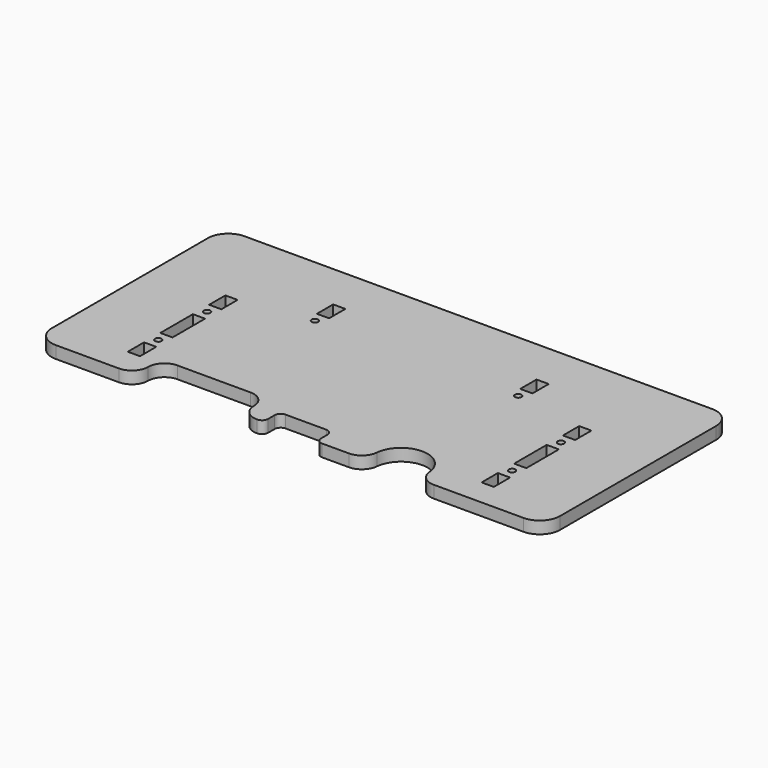
from build123d import *

# Parameters (mm, degrees)
F0_W     = 250
F0_H     = 116
F1_DEPTH = 6
F2_W     = 6
F2_H     = 10
F2_H_2   = 20
F2_W_2   = 26
F2_R     = 1.6
F2_W_3   = 52
F2_H_3   = 16
F3_DEPTH = 6.001
F4_R     = 3
F5_R     = 10
F6_R     = 7.99999
F7_R     = 1.6
F7_W     = 6
F7_H     = 10
F8_DEPTH = 6.0010001


# Not quite as in the source:
# - a fillet or chamfer is up to 0.001 mm smaller than in the source, because OpenCascade refuses the exact size


with BuildPart() as f1:
    # F0 (on Top) → F1 (new body)
    with BuildSketch(Plane.XY):
        Rectangle(F0_W, F0_H)
    extrude(amount=F1_DEPTH)

    # F2 (on face) → F3 (cut, through all)
    with BuildSketch(Plane.XY.offset(6)):
        with Locations((-87, -40)):
            Rectangle(F2_W, F2_H)
        with Locations((-87, 10)):
            Rectangle(F2_W, F2_H)
        with Locations((87, -40)):
            Rectangle(F2_W, F2_H)
        with Locations((87, 10)):
            Rectangle(F2_W, F2_H)
        with Locations((-87, -15)):
            Rectangle(F2_W, F2_H_2)
        with Locations((87, -15)):
            Rectangle(F2_W, F2_H_2)
        with Locations((0, -53)):
            Rectangle(F2_W_2, F2_H)
        with Locations((-87, -30)):
            Circle(F2_R)
        with Locations((-87, 0)):
            Circle(F2_R)
        with Locations((87, -30)):
            Circle(F2_R)
        with Locations((87, 0)):
            Circle(F2_R)
        with BuildLine():
            Line((37, -58), (63, -58))
            Line((63, -58), (63, -52))
            ThreePointArc((63, -52), (50, -39), (37, -52))
            Line((37, -52), (37, -58))
        make_face()
        with Locations((-50, -50)):
            Rectangle(F2_W_3, F2_H_3)
    extrude(amount=-F3_DEPTH, mode=Mode.SUBTRACT)

    # F4
    f4_edges = [f1.edges().sort_by_distance(p)[0] for p in [
        (-13, -48, 3),
        (13, -48, 3),
        (-13, -58, 3),
        (13, -58, 3),
    ]]
    fillet(f4_edges, radius=F4_R)

    # F5
    f5_edges = [f1.edges().sort_by_distance(p)[0] for p in [
        (-125, -58, 3),
        (125, -58, 3),
        (125, 58, 3),
        (-125, 58, 3),
    ]]
    fillet(f5_edges, radius=F5_R)

    # F6 (radius 8 in the source; OpenCascade refuses exactly that, so slightly less here)
    f6_edges = [f1.edges().sort_by_distance(p)[0] for p in [
        (37, -58, 3),
        (63, -58, 3),
        (-24, -58, 3),
        (-24, -42, 3),
        (-76, -42, 3),
        (-76, -58, 3),
    ]]
    fillet(f6_edges, radius=F6_R)

    # F7 (on face) → F8 (cut, through all)
    with BuildSketch(Plane.XY.offset(6)):
        with Locations((-50, 20)):
            Circle(F7_R)
        with Locations((-50, 30)):
            Rectangle(F7_W, F7_H)
        with Locations((50, 30)):
            Rectangle(F7_W, F7_H)
        with Locations((50, 20)):
            Circle(F7_R)
    extrude(amount=-F8_DEPTH, mode=Mode.SUBTRACT)


solid = f1.part
